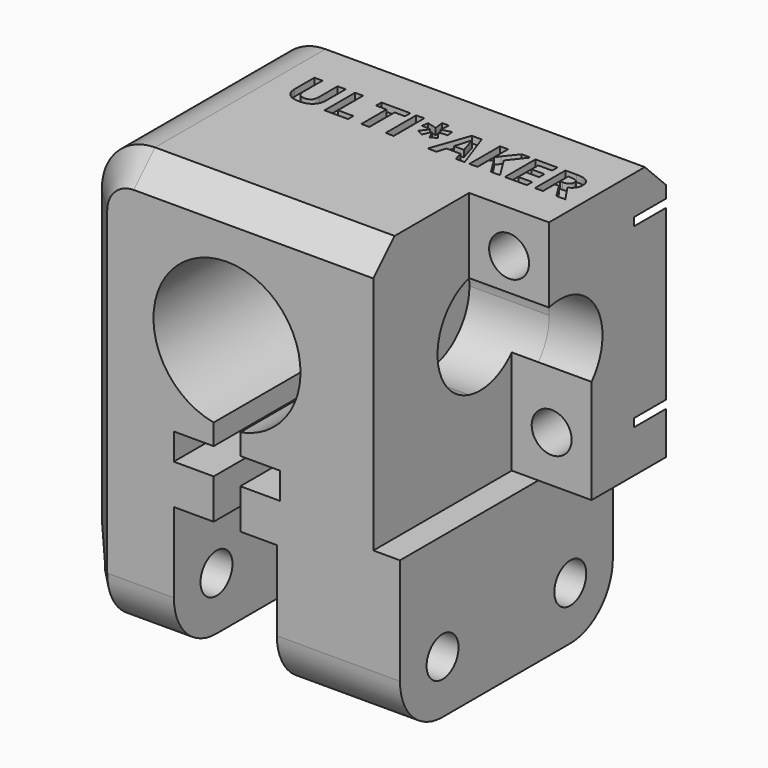
from build123d import *
from build123d import SkipClean  # not in build123d's __all__

# Parameters (mm, degrees)
F0_W           = 24
F0_H           = 32
F1_DEPTH       = 20
F2_W           = 2
F2_H           = 20
F3_DEPTH       = 9
F4_R           = 5.525
F5_DEPTH       = 25
F7_DEPTH       = 25
F8_R           = 1.5
F9_DEPTH       = 25
F11_DEPTH      = 6
F12_W          = 13
F12_H          = 8.4217982061
F13_DEPTH      = 25
F15_DEPTH      = 4
F16_R          = 1.5
F17_DEPTH      = 12.5
F19_DEPTH      = 3
F21_DEPTH      = 3
F22_R          = 4
F23_T1_DEPTH   = 23.1433659759
F23_T3_DEPTH   = 24
F23_T5_DEPTH   = 12
F23_T7_DEPTH   = 29.1433659759
F23_T10_ANGLE  = 90
F23_T12_ANGLE  = 90
F23_T14_ANGLE  = 90
F23_T16_ANGLE  = 90
F24_TEXT_SIZE  = 4.0187611553
F25_DEPTH      = 0.5
F27_DEPTH      = 3
F27_DEPTH_BACK = 5


# Not quite as in the source:
# - a fillet or chamfer that OpenCascade refuses, or shapes differently, is made with other operations: its cross-section is extruded or revolved along the edge and cut away or added
# - after a boolean that leaves OpenCascade's solid faulty, fix() repairs it
# - Text() gives the source's letters only with a copy of the font that has no kerning and outlines rounded to 1/6400 em; it was checked with that copy


with BuildPart() as f1:
    # F0 (on Front) → F1 (new body)
    with BuildSketch(Plane.XZ):
        with Locations((12, 16)):
            Rectangle(F0_W, F0_H)
    extrude(amount=F1_DEPTH)

    # F2 (on face) → F3 (cut)
    with BuildSketch(Plane.XZ.offset(20)):
        with Locations((23, 22)):
            Rectangle(F2_W, F2_H)
    extrude(amount=-F3_DEPTH, mode=Mode.SUBTRACT)

    # F4 (on face) → F5 (cut)
    with BuildSketch(Plane.XZ.offset(20)):
        with Locations((11, 22)):
            Circle(F4_R)
    extrude(amount=-F5_DEPTH, mode=Mode.SUBTRACT)

    # F6 (on face) → F7 (cut)
    with BuildSketch(Plane.XZ.offset(20)):
        Polygon((12, 20.1657801984), (10, 20.1657801984), (10, 10), (7.0111590475, 10), (7.0111590475, -0.1657801984), (10, -0.1657801984), (12, -0.1657801984), (14.75, -0.1657801984), (14.75, 10), (12, 10), align=None)
    extrude(amount=-F7_DEPTH, mode=Mode.SUBTRACT)

    # F8 (on face) → F9 (cut)
    with BuildSketch(Plane.YZ.offset(24)):
        with Locations((-16, 4)):
            Circle(F8_R)
        with Locations((-4, 4)):
            Circle(F8_R)
    extrude(amount=-F9_DEPTH, mode=Mode.SUBTRACT)

    # F10 (on face) → F11 (cut)
    with BuildSketch(Plane.YZ.offset(24)):
        with BuildLine():
            Line((-11, 18.6339293632), (-11, 26.3660706368))
            ThreePointArc((-11, 26.3660706368), (-13.9735995755, 22.5), (-11, 18.6339293632))
        make_face()
        with BuildLine():
            ThreePointArc((-11, 18.6339293632), (-7.5349115776, 19.3293847838), (-5.9735995755, 22.5))
            ThreePointArc((-5.9735995755, 22.5), (-7.5349115776, 25.6706152162), (-11, 26.3660706368))
            Line((-11, 26.3660706368), (-11, 18.6339293632))
        make_face()
    extrude(amount=-F11_DEPTH, mode=Mode.SUBTRACT)

    # F12 (on face) → F13 (cut)
    with BuildSketch(Plane.YZ.offset(22)):
        with Locations((-13.5, 16.2108991031)):
            Rectangle(F12_W, F12_H)
    extrude(amount=F13_DEPTH, mode=Mode.SUBTRACT)

    # F14 (on face) → F15 (join)
    with BuildSketch(Plane.YZ.offset(24)):
        with BuildLine():
            Line((-7, 19.8246111376), (-7, 12))
            Line((-7, 12), (0, 12))
            Line((0, 12), (0, 23.4263278544))
            Line((0, 23.4263278544), (0, 32))
            Line((0, 32), (-7, 32))
            Line((-7, 32), (-11, 32))
            Line((-11, 32), (-11, 26.3660706368))
            ThreePointArc((-11, 26.3660706368), (-6.5610390664, 24.5867272874), (-7, 19.8246111376))
        make_face()
    with SkipClean():  # cleaning this boolean's faces spoils the solid; the shape is the same uncleaned
        extrude(amount=F15_DEPTH)

    # F16 (on face) → F17 (cut, symmetric)
    with BuildSketch(Plane.XZ.offset(7)):
        with Locations((25, 15.5)):
            Circle(F16_R)
        with Locations((25, 28.8)):
            Circle(F16_R)
    extrude(amount=F17_DEPTH, both=True, mode=Mode.SUBTRACT)

    add(f1.part.fix(), mode=Mode.REPLACE)

    # F18 (on face) → F19 (cut)
    with BuildSketch(Plane(origin=(0, 0, 0), x_dir=(-1, 0, 0), z_dir=(0, 1, 0))):
        Polygon((-28.1754264805, 28.8), (-26.5877132403, 26.05), (-23.4122867597, 26.05), (-21.8245735195, 28.8), (-23.4122867597, 31.55), (-26.5877132403, 31.55), align=None)
        Polygon((-26.5877132403, 18.25), (-28.1754264805, 15.5), (-26.5877132403, 12.75), (-23.4122867597, 12.75), (-21.8245735195, 15.5), (-23.4122867597, 18.25), align=None)
    extrude(amount=-F19_DEPTH, mode=Mode.SUBTRACT)

    # F20 (on face) → F21 (cut)
    with BuildSketch(Plane(origin=(0, 0, 0), x_dir=(0, -1, 0), z_dir=(-1, 0, 0))):
        Polygon((5.5877132403, 6.75), (2.4122867597, 6.75), (0.8245735195, 4), (2.4122867597, 1.25), (5.5877132403, 1.25), (7.1754264805, 4), align=None)
        Polygon((17.5877132403, 6.75), (14.4122867597, 6.75), (12.8245735195, 4), (14.4122867597, 1.25), (17.5877132403, 1.25), (19.1754264805, 4), align=None)
    extrude(amount=-F21_DEPTH, mode=Mode.SUBTRACT)

    # F22
    f22_edges = [f1.edges().sort_by_distance(p)[0] for p in [
        (0, -10, 32),
        (3.50558, -20, 0),
        (3.50558, 0, 0),
        (19.375, 0, 0),
        (19.375, -20, 0),
    ]]
    fillet(f22_edges, radius=F22_R)

    # F23: chamfer of 2 on 2 edges, made by hand

    # F23_s2 → F23_t1 (cut)
    with BuildSketch(Plane.YZ.offset(4)):
        Polygon((-20, 30), (-18, 32), (-20, 32), align=None)
    extrude(amount=F23_T1_DEPTH, mode=Mode.SUBTRACT)

    # F23_s4 → F23_t3 (cut)
    with BuildSketch(Plane.XY.offset(4)):
        Polygon((0, -18), (2, -20), (0, -20), align=None)
        Polygon((0, -2), (2, 0), (0, 0), align=None)
    extrude(amount=F23_T3_DEPTH, mode=Mode.SUBTRACT)

    # F23_s6 → F23_t5 (cut)
    with BuildSketch(Plane.XZ.offset(4)):
        Polygon((0, 2), (2, 0), (0, 0), align=None)
    extrude(amount=F23_T5_DEPTH, mode=Mode.SUBTRACT)

    # F23_s8 → F23_t7 (cut)
    with BuildSketch(Plane.YZ.offset(4)):
        Polygon((0, 30), (-2, 32), (0, 32), align=None)
    extrude(amount=F23_T7_DEPTH, mode=Mode.SUBTRACT)

    # F23_s9 → F23_t10 (revolve, cut)
    with BuildSketch(Plane.XY.offset(28)):
        Polygon((0, -18), (2, -20), (0, -20), align=None)
    revolve(axis=Axis((4, -20, 28), (0, 1, 0)), revolution_arc=F23_T10_ANGLE, mode=Mode.SUBTRACT)

    # F23_s11 → F23_t12 (revolve, cut)
    with BuildSketch(Plane.XY.offset(4)):
        Polygon((0, -18), (2, -20), (0, -20), align=None)
    revolve(axis=Axis((0, -16, 4), (1, 0, 0)), revolution_arc=F23_T12_ANGLE, mode=Mode.SUBTRACT)

    # F23_s13 → F23_t14 (revolve, cut)
    with BuildSketch(Plane.XY.offset(4)):
        Polygon((0, -2), (2, 0), (0, 0), align=None)
    revolve(axis=Axis((0, -4, 4), (-1, 0, 0)), revolution_arc=F23_T14_ANGLE, mode=Mode.SUBTRACT)

    # F23_s15 → F23_t16 (revolve, cut)
    with BuildSketch(Plane.XY.offset(28)):
        Polygon((2, 0), (0, -2), (0, 0), align=None)
    revolve(axis=Axis((4, 0, 28), (0, 1, 0)), revolution_arc=F23_T16_ANGLE, mode=Mode.SUBTRACT)

    # F24 (on face) → F25 (cut)
    with BuildSketch(Plane.XY.offset(32)):
        with Locations((5.4171234369, -8.1119630486)):
            Text('ULTI*AKER', F24_TEXT_SIZE, font='Open Sans', font_style=FontStyle.BOLD, text_align=(TextAlign.LEFT, TextAlign.BOTTOM))
    extrude(amount=-F25_DEPTH, mode=Mode.SUBTRACT)

    # F26 (on face) → F27 (cut, two sides)
    with BuildSketch(Plane.YZ.offset(10)) as f27_sk:
        with BuildLine():
            Line((-11.8646633625, 11), (-11.8646633625, 10))
            Line((-11.8646633625, 10), (-7.8646633625, 10))
            Line((-7.8646633625, 10), (-7.8646633625, 11))
            ThreePointArc((-7.8646633625, 11), (-7.2788769249, 12.4142135624), (-5.8646633625, 13))
            Line((-5.8646633625, 13), (0, 13))
            Line((0, 13), (0, 15))
            Line((0, 15), (-7.8646633625, 15))
            Line((-7.8646633625, 15), (-11.8646633625, 15))
            Line((-11.8646633625, 15), (-20, 15))
            Line((-20, 15), (-20, 13))
            Line((-20, 13), (-13.8646633625, 13))
            ThreePointArc((-13.8646633625, 13), (-12.4504498001, 12.4142135624), (-11.8646633625, 11))
        make_face()
    extrude(amount=-F27_DEPTH, mode=Mode.SUBTRACT)
    extrude(f27_sk.sketch, amount=F27_DEPTH_BACK, mode=Mode.SUBTRACT)


solid = f1.part
